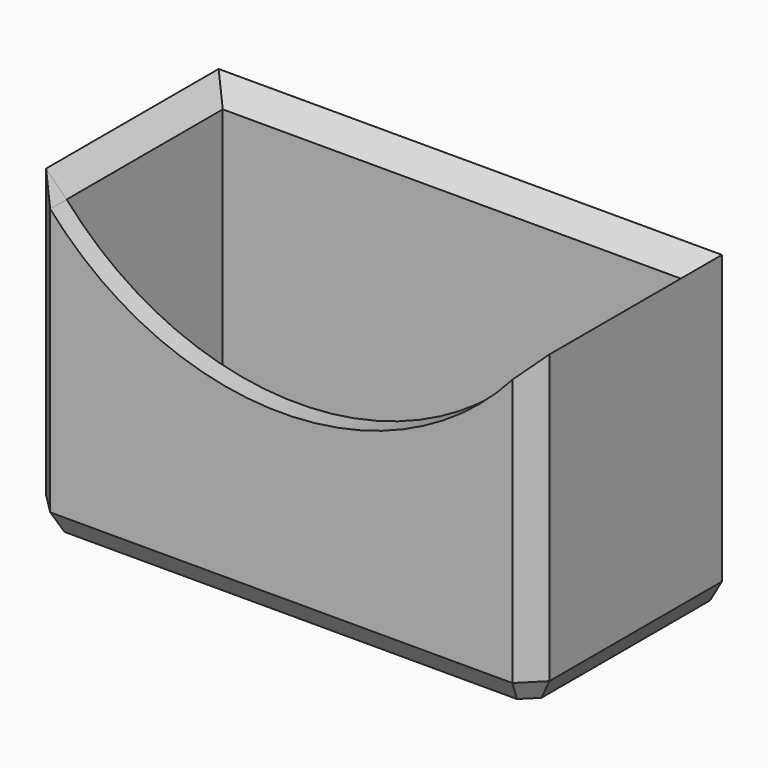
from build123d import *

# Parameters (mm, degrees)
F0_W     = 49
F0_H     = 23
F1_DEPTH = 30
F2_T     = -2
F3_SIZE  = 1.99999
F5_DEPTH = 2
F6_SIZE  = 1.9999
F7_SIZE  = 1.99999
F8_SIZE2 = 1.1547005384
F8_SIZE  = 2


# Not quite as in the source:
# - a fillet or chamfer is up to 0.001 mm smaller than in the source, because OpenCascade refuses the exact size


with BuildPart() as f1:
    # F0 (on Top) → F1 (new body)
    with BuildSketch(Plane.XY):
        Rectangle(F0_W, F0_H)
    extrude(amount=F1_DEPTH)

    # F2
    f2_openings = [f1.faces().sort_by_distance(p)[0] for p in [
        (0, 0, 30),
    ]]
    offset(amount=F2_T, openings=f2_openings)

    # F3 (size 2 in the source; OpenCascade refuses exactly that, so slightly less here)
    f3_edges = [f1.edges().sort_by_distance(p)[0] for p in [
        (0, 9.5, 30),
        (-22.5, 0, 30),
        (22.5, 0, 30),
    ]]
    chamfer(f3_edges, length=F3_SIZE)

    # F4 (on face) → F5 (cut, through all)
    with BuildSketch(Plane.XZ.offset(11.5)):
        with BuildLine():
            Line((-22.5, 30), (-22.5, 28))
            ThreePointArc((-22.5, 28), (0, 17.843134833), (22.5, 28))
            Line((22.5, 28), (22.5, 30))
            Line((22.5, 30), (-22.5, 30))
        make_face()
    extrude(amount=-F5_DEPTH, mode=Mode.SUBTRACT)

    # F6 (size 2 in the source; OpenCascade refuses exactly that, so slightly less here)
    f6_edges = [f1.edges().sort_by_distance(p)[0] for p in [
        (-22.5, -10.5, 30),
        (22.5, -10.5, 30),
    ]]
    chamfer(f6_edges, length=F6_SIZE)

    # F7 (size 2 in the source; OpenCascade refuses exactly that, so slightly less here)
    f7_edges = [f1.edges().sort_by_distance(p)[0] for p in [
        (-24.5, -11.5, 15),
        (24.5, -11.5, 15),
    ]]
    chamfer(f7_edges, length=F7_SIZE)

    # F8
    f8_edges = [f1.edges().sort_by_distance(p)[0] for p in [
        (24.5, 0.999995, 0),
        (23.500005, -10.500005, 0),
        (0, -11.5, 0),
        (-23.500005, -10.500005, 0),
        (-24.5, 0.999995, 0),
    ]]
    chamfer(f8_edges, length=F8_SIZE, length2=F8_SIZE2)


solid = f1.part
